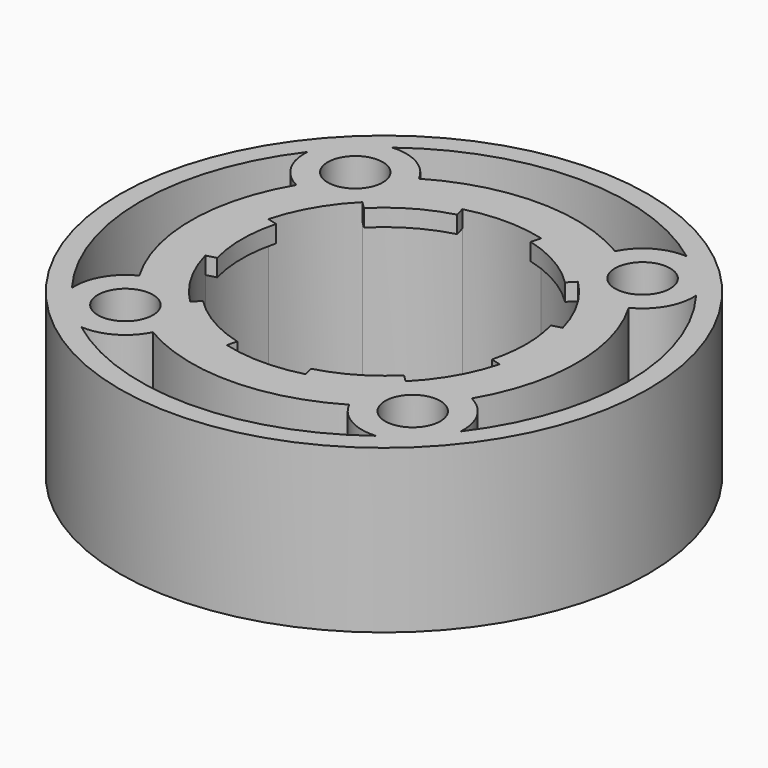
from build123d import *

# Parameters (mm, degrees)
F0_R            = 20.6375
F0_R_2          = 2.15265
F1_DEPTH        = 12.7
F3_DEPTH        = 12.7
F4_COUNT        = 6
F4_ANGLE        = 300
F6_R            = 11.90625
F7_DEPTH        = 11.36015
F9_DEPTH        = 12.7
F9_COPIES_COUNT = 4


# Not quite as in the source:
# - a pattern or mirror of a feature is missing from the dataset's text; its kind, count and spacing are read off the source's solid


with BuildPart() as f1:
    # F0 (on Top) → F1 (new body)
    with BuildSketch(Plane.XY):
        Circle(F0_R)
        with Locations((-11.2253201513, -11.2253201513)):
            Circle(F0_R_2, mode=Mode.SUBTRACT)
        with Locations((11.2253201513, -11.2253201513)):
            Circle(F0_R_2, mode=Mode.SUBTRACT)
        with Locations((-11.2253201513, 11.2253201513)):
            Circle(F0_R_2, mode=Mode.SUBTRACT)
        with BuildLine():
            ThreePointArc((0, 11.1125), (7.8577241059, 7.8577241059), (11.1125, 0))
            ThreePointArc((11.1125, 0), (-7.8577241059, -7.8577241059), (0, 11.1125))
        make_face(mode=Mode.SUBTRACT)
        with Locations((11.2253201513, 11.2253201513)):
            Circle(F0_R_2, mode=Mode.SUBTRACT)
    extrude(amount=F1_DEPTH)

    # F2 (on face) → F3 (cut, through all)
    with BuildSketch(Plane.XY.offset(12.7)):
        with BuildLine():
            ThreePointArc((-2.8761266387, 10.7338507446), (0, 11.1125), (2.8761266387, 10.7338507446))
            Line((2.8761266387, 10.7338507446), (3.0815642558, 11.5005543693))
            ThreePointArc((3.0815642558, 11.5005543693), (0, 11.90625), (-3.0815642558, 11.5005543693))
            Line((-3.0815642558, 11.5005543693), (-2.8761266387, 10.7338507446))
        make_face()
    f3 = extrude(amount=-F3_DEPTH, mode=Mode.SUBTRACT)

    # F4: F3 ×6 about axis
    f4_axis = Axis((0, 0, 0), (0, 0, -1))
    for i in range(1, F4_COUNT):
        add(f3.rotate(f4_axis, i * F4_ANGLE / (F4_COUNT - 1)), mode=Mode.SUBTRACT)

    # F6 (on face) → F7 (cut, through all)
    with BuildSketch(Plane(origin=(0, 0, 0), x_dir=(1, 0, 0), z_dir=(0, 0, -1))):
        Circle(F6_R)
    extrude(amount=-F7_DEPTH, mode=Mode.SUBTRACT)

    # F8 (on face) → F9 (cut, through all)
    with BuildSketch(Plane(origin=(0, 0, 0), x_dir=(1, 0, 0), z_dir=(0, 0, -1))):
        with BuildLine():
            ThreePointArc((11.5039191556, -15.1842795042), (9.251826165, -14.6686177057), (7.6685282311, -12.9860608474))
            ThreePointArc((7.6685282311, -12.9860608474), (0, -15.08125), (-7.6685282311, -12.9860608474))
            ThreePointArc((-7.6685282311, -12.9860608474), (-9.251826165, -14.6686177057), (-11.5039191556, -15.1842795042))
            ThreePointArc((-11.5039191556, -15.1842795042), (0, -19.05), (11.5039191556, -15.1842795042))
        make_face()
    f9 = extrude(amount=-F9_DEPTH, mode=Mode.SUBTRACT)

    # F9_copies: F9 ×4 about axis
    f9_copies_axis = Axis((0, 0, 0), (0, 0, 1))
    for i in range(1, F9_COPIES_COUNT):
        add(f9.rotate(f9_copies_axis, i * 360 / F9_COPIES_COUNT), mode=Mode.SUBTRACT)


solid = f1.part
